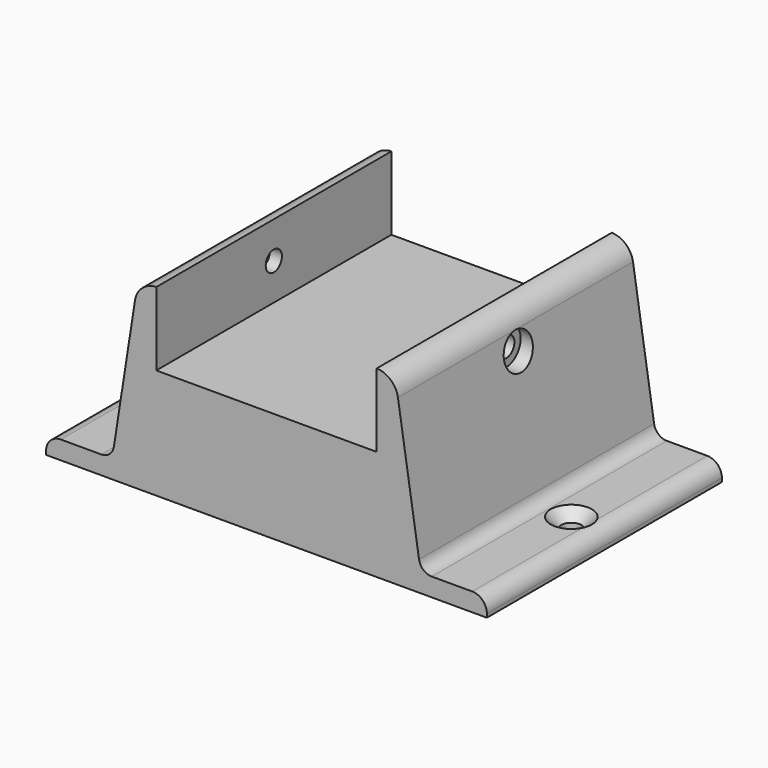
from build123d import *

# Parameters (mm, degrees)
F1_DEPTH              = 80
F10_D                 = 5.5
F10_DEPTH             = 10
F10_CSINK_D           = 11.2
F10_CSINK_ANGLE       = 90
F10_TIP               = 1.6523667023
F10_ON_F3_D           = 5.5
F10_ON_F3_DEPTH       = 10
F10_ON_F3_CSINK_D     = 11.2
F10_ON_F3_CSINK_ANGLE = 90
F10_ON_F3_TIP         = 1.6523667023
F11_D                 = 5.5
F11_DEPTH             = 10
F11_START             = 2.7027778
F11_CBORE_D           = 9.75
F11_CBORE_DEPTH       = 2.5
F11_TIP               = 1.6523667023
F12_D                 = 5.5
F12_DEPTH             = 10
F12_START             = 2.7027778
F12_CBORE_D           = 9.75
F12_CBORE_DEPTH       = 2.5
F12_TIP               = 1.6523667023
F13_T1_DEPTH          = 105.6859695087
F14_R                 = 3.5
F15_T1_DEPTH          = 100


# Not quite as in the source:
# - a fillet or chamfer that OpenCascade refuses, or shapes differently, is made with other operations: its cross-section is extruded or revolved along the edge and cut away or added


with BuildPart() as f1:
    # F0 (on Front) → F1 (new body)
    with BuildSketch(Plane.XZ):
        Polygon((-60, 5), (-60, 0), (60, 0), (60, 5), (42, 5), (35, 50), (30, 50), (30, 30), (-30, 30), (-30, 50), (-35, 50), (-42, 5), align=None)
    extrude(amount=F1_DEPTH)

    # F10
    with Locations(Plane.XY.offset(5)):
        with Locations((-51, -40)):
            CounterSinkHole(F10_D / 2, F10_CSINK_D / 2, depth=F10_DEPTH, counter_sink_angle=F10_CSINK_ANGLE)
            with Locations((0, 0, -(F10_DEPTH + F10_TIP / 2))):  # 118° drill point
                Cone(0, F10_D / 2, F10_TIP, mode=Mode.SUBTRACT)

    # F10 on F3
    with Locations(Plane.XY.offset(5)):
        with Locations((51, -40)):
            CounterSinkHole(F10_ON_F3_D / 2, F10_ON_F3_CSINK_D / 2, depth=F10_ON_F3_DEPTH, counter_sink_angle=F10_ON_F3_CSINK_ANGLE)
            with Locations((0, 0, -(F10_ON_F3_DEPTH + F10_ON_F3_TIP / 2))):  # 118° drill point
                Cone(0, F10_ON_F3_D / 2, F10_ON_F3_TIP, mode=Mode.SUBTRACT)

    # F11
    # its depths count from where the whole tool has entered the part; down to there all is cleared
    with Locations(Plane(origin=(-38.5, 0, 0), x_dir=(0, 1, 0), z_dir=(-1, 0, 0)).offset(-F11_START)):
        with Locations((-40, -40)):
            CounterBoreHole(F11_D / 2, F11_CBORE_D / 2, F11_CBORE_DEPTH, depth=F11_DEPTH)
            with Locations((0, 0, -(F11_DEPTH + F11_TIP / 2))):  # 118° drill point
                Cone(0, F11_D / 2, F11_TIP, mode=Mode.SUBTRACT)

    # F12
    # its depths count from where the whole tool has entered the part; down to there all is cleared
    with Locations(Plane.YZ.offset(38.5).offset(-F12_START)):
        with Locations((-40, 40)):
            CounterBoreHole(F12_D / 2, F12_CBORE_D / 2, F12_CBORE_DEPTH, depth=F12_DEPTH)
            with Locations((0, 0, -(F12_DEPTH + F12_TIP / 2))):  # 118° drill point
                Cone(0, F12_D / 2, F12_TIP, mode=Mode.SUBTRACT)

    # F13: fillet of radius 6 on 2 edges, made by hand

    # F13_s2 → F13_t1 (cut)
    with BuildSketch(Plane.XZ.offset(-12.8429847543)):
        with BuildLine():
            ThreePointArc((-35.7896226953, 44.9238541015), (-33.8164627137, 48.513120963), (-30, 50))
            Line((-30, 50), (-35, 50))
            Line((-35, 50), (-35.7896226953, 44.9238541015))
        make_face()
        with BuildLine():
            ThreePointArc((35.7896226953, 44.9238541015), (33.8164627137, 48.513120963), (30, 50))
            Line((30, 50), (35, 50))
            Line((35, 50), (35.7896226953, 44.9238541015))
        make_face()
    extrude(amount=F13_T1_DEPTH, mode=Mode.SUBTRACT)

    # F14
    f14_edges = [f1.edges().sort_by_distance(p)[0] for p in [
        (-42, -40, 5),
        (42, -40, 5),
    ]]
    fillet(f14_edges, radius=F14_R)

    # F15: fillet of radius 4 on 2 edges, made by hand

    # F15_s2 → F15_t1 (cut)
    with BuildSketch(Plane.XZ.offset(-10)):
        with BuildLine():
            ThreePointArc((-56, 5), (-58.8284271247, 3.8284271247), (-60, 1))
            Line((-60, 1), (-60, 5))
            Line((-60, 5), (-56, 5))
        make_face()
        with BuildLine():
            ThreePointArc((60, 1), (58.8284271247, 3.8284271247), (56, 5))
            Line((56, 5), (60, 5))
            Line((60, 5), (60, 1))
        make_face()
    extrude(amount=F15_T1_DEPTH, mode=Mode.SUBTRACT)


solid = f1.part
